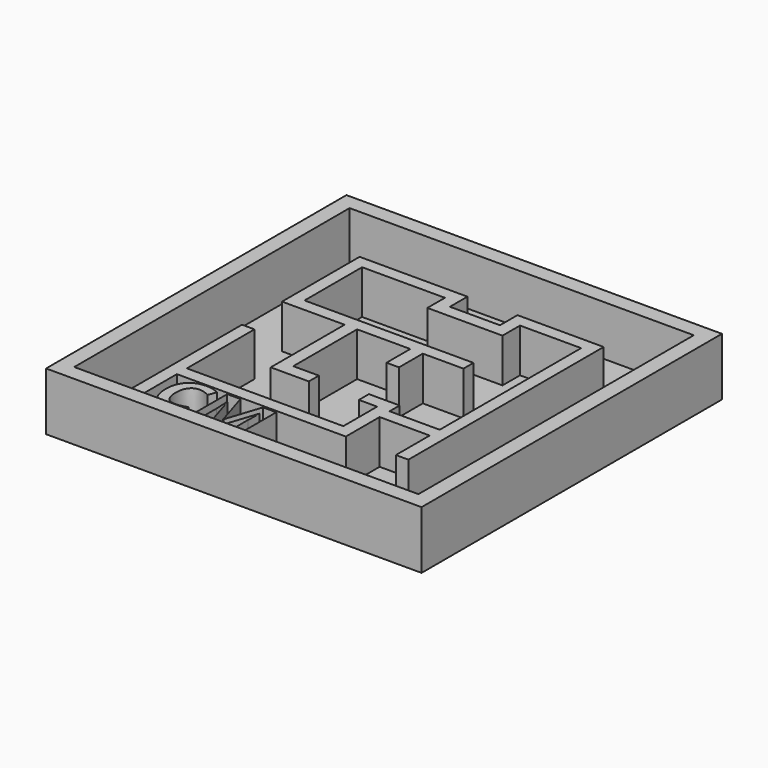
from build123d import *

# Parameters (mm, degrees)
F0_W         = 38.1
F0_H         = 38.1
F1_DEPTH     = 0.79375
F2_W         = 38.1
F2_H         = 38.1
F2_W_2       = 34.925
F2_H_2       = 34.925
F3_DEPTH     = 5.08
F4_W         = 1.27
F4_H         = 1.27
F4_W_2       = 1.8474577538
F4_W_3       = 5.08
F4_W_4       = 0.0586806464
F4_H_2       = 4.445
F4_H_3       = 0.9525
F4_H_4       = 3.01625
F4_TEXT_SIZE = 6.5263888889
F5_DEPTH     = 4.445
F6_R         = 1.27
F7_DEPTH     = 0.396875


# Not quite as in the source:
# - Text() gives the source's letters only with a copy of the font that has no kerning and outlines rounded to 1/6400 em; it was checked with that copy


with BuildPart() as f1:
    # F0 (on Top) → F1 (new body)
    with BuildSketch(Plane.XY):
        with Locations((2.7097854763, -1.968138108)):
            Rectangle(F0_W, F0_H)
    extrude(amount=F1_DEPTH)

    # F2 (on face) → F3 (join)
    with BuildSketch(Plane.XY.offset(0.79375)):
        with Locations((2.7097854763, -1.968138108)):
            Rectangle(F2_W, F2_H)
        with Locations((2.7097854763, -1.968138108)):
            Rectangle(F2_W_2, F2_H_2, mode=Mode.SUBTRACT)
    extrude(amount=F3_DEPTH)

    # F4 (on face) → F5 (join)
    with BuildSketch(Plane.XY.offset(0.79375)):
        Polygon((-9.6727145237, -4.508138108), (-9.6727145237, -19.430638108), (-8.4027145237, -19.430638108), (-8.4027145237, -14.350638108), (-8.4027145237, -13.080638108), (-8.4027145237, -4.508138108), align=None)
        Polygon((-8.4027145237, -13.080638108), (-8.4027145237, -14.350638108), (8.7422854763, -14.350638108), (8.7422854763, -13.080638108), (7.4722854763, -13.080638108), align=None)
        Polygon((7.4722854763, -8.794388108), (7.4722854763, -13.080638108), (8.7422854763, -13.080638108), (8.7422854763, -10.064388108), (8.7422854763, -8.794388108), align=None)
        with Locations((8.1072854763, -8.159388108)):
            Rectangle(F4_W, F4_H)
        with Locations((6.5485565994, -8.159388108)):
            Rectangle(F4_W_2, F4_H)
        with Locations((11.2822854763, -9.429388108)):
            Rectangle(F4_W_3, F4_H)
        Polygon((13.8809661227, -10.064388108), (13.8222854763, -10.064388108), (13.8222854763, -14.350638108), (15.0922854763, -14.350638108), (15.0922854763, -8.000638108), (13.8222854763, -8.000638108), (13.8222854763, -8.794388108), (13.8809661227, -8.794388108), align=None)
        with Locations((13.8516257995, -9.429388108)):
            Rectangle(F4_W_4, F4_H)
        Polygon((13.8222854763, -3.714388108), (13.8222854763, -8.000638108), (15.0922854763, -8.000638108), (15.0922854763, 4.699361892), (13.8222854763, 4.699361892), (13.8222854763, -2.0651470404), align=None)
        with Locations((14.4572854763, 6.921861892)):
            Rectangle(F4_W, F4_H_2)
        Polygon((13.8222854763, 9.144361892), (15.0922854763, 9.144361892), (15.0922854763, 10.414361892), (6.35, 10.414361892), (6.35, 9.144361892), (7.62, 9.144361892), (10.1695209742, 9.144361892), (11.4395209742, 9.144361892), align=None)
        with Locations((6.985, 8.668111892)):
            Rectangle(F4_W, F4_H_3)
        with Locations((3.81, 7.556861892)):
            Rectangle(F4_W_3, F4_H)
        with Locations((6.985, 7.556861892)):
            Rectangle(F4_W, F4_H)
        Polygon((1.27, 6.921861892), (1.27, 8.191861892), (1.27, 9.144361892), (0, 9.144361892), (0, 6.921861892), align=None)
        Polygon((0, 9.144361892), (1.27, 9.144361892), (1.27, 10.414361892), (-8.4027145237, 10.414361892), (-8.4027145237, 9.144361892), (-3.3227145237, 9.144361892), (-2.0527145237, 9.144361892), align=None)
        Polygon((-8.4027145237, 9.144361892), (-8.4027145237, 10.414361892), (-9.6727145237, 10.414361892), (-9.6727145237, 0.571861892), (-8.4027145237, 0.571861892), (-8.4027145237, 1.841861892), align=None)
        Polygon((-2.0527145237, 1.841861892), (-8.4027145237, 1.841861892), (-8.4027145237, 0.571861892), (-3.3227145237, 0.571861892), (-2.0527145237, 0.571861892), align=None)
        Polygon((-0.7129738806, 1.841861892), (-2.0527145237, 1.841861892), (-2.0527145237, 0.571861892), (3.3447854763, 0.571861892), (4.6147854763, 0.571861892), (8.7422854763, 0.571861892), (8.7422854763, 1.841861892), (0.5570261194, 1.841861892), align=None)
        Polygon((-2.0527145237, 0.571861892), (-3.3227145237, 0.571861892), (-3.3227145237, -7.524388108), (-2.426698155, -7.524388108), (-2.0527145237, -7.524388108), (-2.0527145237, -3.714388108), (-2.0527145237, -2.0651470404), align=None)
        Polygon((-2.426698155, -7.524388108), (-3.3227145237, -7.524388108), (-3.3227145237, -8.000638108), (-2.0527145237, -8.000638108), (-2.0527145237, -7.524388108), align=None)
        with Locations((3.9797854763, -0.936263108)):
            Rectangle(F4_W, F4_H_4)
        Polygon((-2.0527145237, -8.000638108), (-3.3227145237, -8.000638108), (-3.3227145237, -8.794388108), (-2.426698155, -8.794388108), (0.5448277225, -8.794388108), (0.5448277225, -7.524388108), (-2.0527145237, -7.524388108), align=None)
        with Locations((-7.8873597085, -19.2010922646)):
            Text('CM', F4_TEXT_SIZE, font='Open Sans', font_style=FontStyle.BOLD, text_align=(TextAlign.LEFT, TextAlign.BOTTOM))
    extrude(amount=F5_DEPTH)

    # F6 (on face) → F7 (cut)
    with BuildSketch(Plane.XY.offset(0.79375)):
        with Locations((-6.362576969, 7.2121419944)):
            Circle(F6_R)
        with Locations((-12.2127145237, -17.3991657794)):
            Circle(F6_R)
    extrude(amount=-F7_DEPTH, mode=Mode.SUBTRACT)


solid = f1.part
